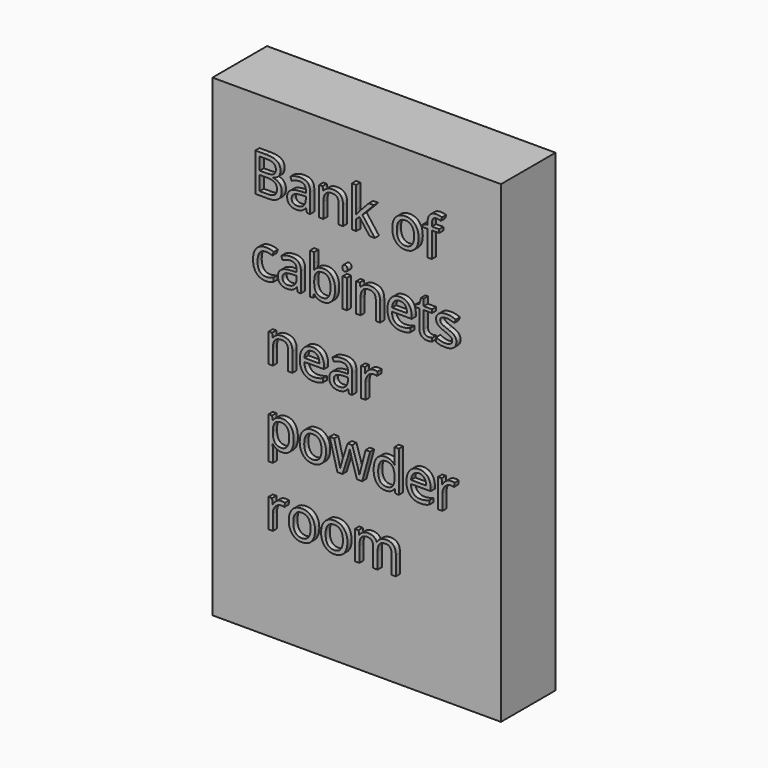
from build123d import *

# Parameters (mm, degrees)
F0_W         = 1397
F0_H         = 2292.35
F1_DEPTH     = 330.2
F2_TEXT_SIZE = 259.0700824734
F3_DEPTH     = 25.4


# Not quite as in the source:
# - Text() gives the source's letters only with a copy of the font that has no kerning and outlines rounded to 1/6400 em; it was checked with that copy


with BuildPart() as f1:
    # F0 (on Front) → F1 (new body)
    with BuildSketch(Plane.XZ):
        with Locations((-632.6230913997, 1115.6660328835)):
            Rectangle(F0_W, F0_H)
    extrude(amount=F1_DEPTH)

    # F2 (on face) → F3 (join)
    with BuildSketch(Plane.XZ.offset(330.2)):
        with Locations((-1128.9324393715, 1850.4926394195)):
            Text('Bank of', F2_TEXT_SIZE, font='Open Sans', text_align=(TextAlign.LEFT, TextAlign.BOTTOM))
        with Locations((-1128.9324393715, 1498.1573272557)):
            Text('cabinets', F2_TEXT_SIZE, font='Open Sans', text_align=(TextAlign.LEFT, TextAlign.BOTTOM))
        with Locations((-1061.6146976288, 1145.8220150918)):
            Text('near', F2_TEXT_SIZE, font='Open Sans', text_align=(TextAlign.LEFT, TextAlign.BOTTOM))
        with Locations((-1061.6146976288, 793.486702928)):
            Text('powder', F2_TEXT_SIZE, font='Open Sans', text_align=(TextAlign.LEFT, TextAlign.BOTTOM))
        with Locations((-1061.6146976288, 441.1513907642)):
            Text('room', F2_TEXT_SIZE, font='Open Sans', text_align=(TextAlign.LEFT, TextAlign.BOTTOM))
    extrude(amount=F3_DEPTH)


solid = f1.part
